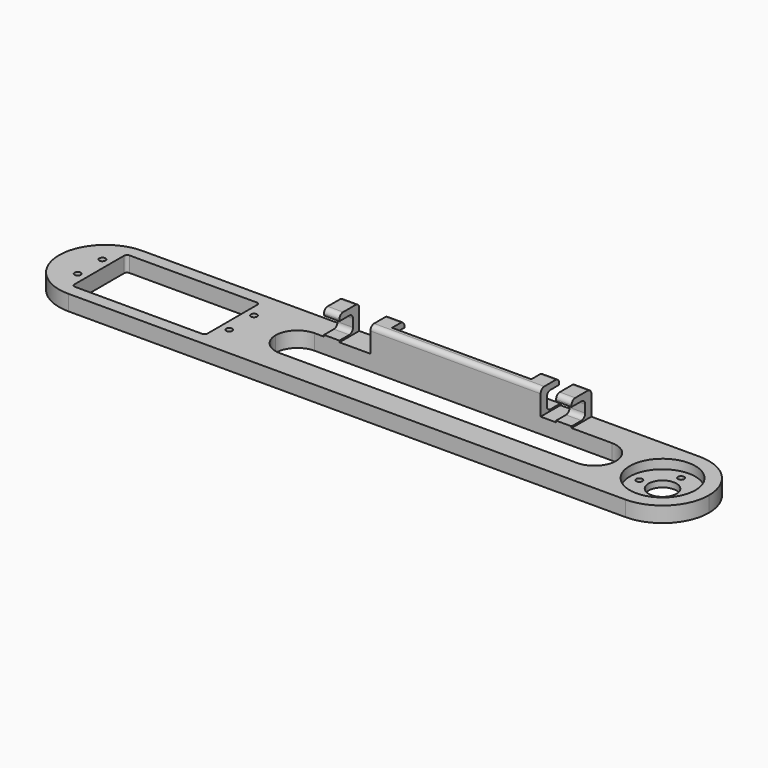
from build123d import *

# Parameters (mm, degrees)
F0_W      = 210
F0_H      = 30
F0_W_2    = 110
F0_H_2    = 14
F1_DEPTH  = 5
F2_R      = 10.6
F2_R_2    = 1
F2_R_3    = 4.5
F2_W      = 43
F2_H      = 22
F2_R_4    = 2.75
F3_DEPTH  = 3
F4_DEPTH  = 25
F5_R      = 14.99999
F6_R      = 6.99999
F7_R      = 1
F8_DEPTH  = 25
F9_W      = 5
F9_H      = 8
F10_DEPTH = 8
F11_W     = 5.5
F11_H     = 5.5
F12_DEPTH = 6
F13_W     = 5.5
F13_H     = 5.5
F14_DEPTH = 6
F15_W     = 5.5
F15_H     = 5.5
F16_W     = 5.5
F16_H     = 5.5
F17_DEPTH = 6
F9_W_2    = 45
F9_H_2    = 2.5
F18_DEPTH = 8
F19_DEPTH = 0.5
F20_R     = 1.5


# Not quite as in the source:
# - a fillet or chamfer is up to 0.001 mm smaller than in the source, because OpenCascade refuses the exact size
# - a feature names something its author has since deleted; it is built from what else it names


with BuildPart() as f1:
    # F0 (on Top) → F1 (new body)
    with BuildSketch(Plane.XY):
        with Locations((-5, -11.8972941886)):
            Rectangle(F0_W, F0_H)
        with Locations((15, -11.8972941886)):
            Rectangle(F0_W_2, F0_H_2, mode=Mode.SUBTRACT)
    extrude(amount=F1_DEPTH)

    # F2 (on face) → F3 (cut)
    with BuildSketch(Plane.XY.offset(5)):
        with Locations((85, -11.8972941886)):
            Circle(F2_R)
        with Locations((85, -19.3972941886)):
            Circle(F2_R_2, mode=Mode.SUBTRACT)
        with Locations((85, -11.8972941886)):
            Circle(F2_R_3, mode=Mode.SUBTRACT)
        with Locations((77.5, -11.8972941886)):
            Circle(F2_R_2, mode=Mode.SUBTRACT)
        with Locations((92.5, -11.8972941886)):
            Circle(F2_R_2, mode=Mode.SUBTRACT)
        with Locations((85, -4.3972941886)):
            Circle(F2_R_2, mode=Mode.SUBTRACT)
        with Locations((-75.5, -11.8972941886)):
            Rectangle(F2_W, F2_H)
        with Locations((-65, -11.8972941886)):
            Circle(F2_R_4, mode=Mode.SUBTRACT)
    extrude(amount=-F3_DEPTH, mode=Mode.SUBTRACT)

    # F2 (on face) → F4 (cut)
    with BuildSketch(Plane.XY.offset(5)):
        with Locations((-75.5, -11.8972941886)):
            Rectangle(F2_W, F2_H)
        with Locations((-65, -11.8972941886)):
            Circle(F2_R_4, mode=Mode.SUBTRACT)
        with Locations((85, -11.8972941886)):
            Circle(F2_R_3)
        with Locations((-65, -11.8972941886)):
            Circle(F2_R_4)
        with Locations((85, -4.3972941886)):
            Circle(F2_R_2)
        with Locations((77.5, -11.8972941886)):
            Circle(F2_R_2)
        with Locations((85, -19.3972941886)):
            Circle(F2_R_2)
        with Locations((92.5, -11.8972941886)):
            Circle(F2_R_2)
    extrude(amount=-F4_DEPTH, mode=Mode.SUBTRACT)

    # F5 (radius 15 in the source; OpenCascade refuses exactly that, so slightly less here)
    f5_edges = [f1.edges().sort_by_distance(p)[0] for p in [
        (100, 3.102706, 2.5),
        (100, -26.897294, 2.5),
        (-110, -26.897294, 2.5),
        (-110, 3.102706, 2.5),
    ]]
    fillet(f5_edges, radius=F5_R)

    # F6 (radius 7 in the source; OpenCascade refuses exactly that, so slightly less here)
    f6_edges = [f1.edges().sort_by_distance(p)[0] for p in [
        (-40, -4.897294, 2.5),
        (-40, -18.897294, 2.5),
        (70, -4.897294, 2.5),
        (70, -18.897294, 2.5),
    ]]
    fillet(f6_edges, radius=F6_R)

    # F7
    f7_edges = [f1.edges().sort_by_distance(p)[0] for p in [
        (-97, -0.897294, 2.5),
        (-97, -22.897294, 2.5),
        (-54, -0.897294, 2.5),
        (-54, -22.897294, 2.5),
    ]]
    fillet(f7_edges, radius=F7_R)

    # F2 (on face) → F8 (cut)
    with BuildSketch(Plane.XY.offset(5)):
        with Locations((-100, -6.8972941886)):
            Circle(F2_R_2)
        with Locations((-100, -16.8972941886)):
            Circle(F2_R_2)
        with Locations((-51, -6.8972941886)):
            Circle(F2_R_2)
        with Locations((-51, -16.8972941886)):
            Circle(F2_R_2)
    extrude(amount=-F8_DEPTH, mode=Mode.SUBTRACT)

    # F9 (on face) → F10 (join)
    with BuildSketch(Plane.XY.offset(5)):
        with Locations((-27.5, -0.8972941886)):
            Rectangle(F9_W, F9_H)
        Polygon((-10, 3.1027058114), (-15, 3.1027058114), (-15, -4.8972941886), (-10, -4.8972941886), (-10, -2.3972941886), align=None)
        Polygon((40, 3.1027058114), (35, 3.1027058114), (35, -2.3972941886), (35, -4.8972941886), (40, -4.8972941886), align=None)
        with Locations((47.5, -0.8972941886)):
            Rectangle(F9_W, F9_H)
    extrude(amount=F10_DEPTH)

    # F11 (on face) → F12 (cut)
    with BuildSketch(Plane(origin=(-30, 0, 0), x_dir=(0, -1, 0), z_dir=(-1, 0, 0))):
        with Locations((2.1472941886, 8.25)):
            Rectangle(F11_W, F11_H)
    extrude(amount=-F12_DEPTH, mode=Mode.SUBTRACT)

    # F13 (on face) → F14 (cut)
    with BuildSketch(Plane(origin=(-15, 0, 0), x_dir=(0, -1, 0), z_dir=(-1, 0, 0))):
        with Locations((-0.3527058114, 8.25)):
            Rectangle(F13_W, F13_H)
    extrude(amount=-F14_DEPTH, mode=Mode.SUBTRACT)

    # F15 (on face) + F16 (on face) → F17 (cut)
    with BuildSketch(Plane(origin=(35, 0, 0), x_dir=(0, -1, 0), z_dir=(-1, 0, 0))):
        with Locations((-0.3527058114, 8.25)):
            Rectangle(F15_W, F15_H)
    with BuildSketch(Plane(origin=(45, 0, 0), x_dir=(0, -1, 0), z_dir=(-1, 0, 0))):
        with Locations((2.1472941886, 8.25)):
            Rectangle(F16_W, F16_H)
    extrude(amount=-F17_DEPTH, mode=Mode.SUBTRACT)

    # F9 (on face) → F18 (join)
    with BuildSketch(Plane.XY.offset(5)):
        with Locations((12.5, -3.6472941886)):
            Rectangle(F9_W_2, F9_H_2)
    extrude(amount=F18_DEPTH)

    # F19 (cut): faces of the model
    f19_faces = [f1.faces().sort_by_distance(p)[0] for p in [
        (37.5, 3.1027058114, 12),
        (-12.5, 3.1027058114, 12),
        (47.5, -4.8972941886, 12),
        (-27.5, -4.8972941886, 12),
    ]]
    extrude(f19_faces, amount=-F19_DEPTH, dir=(0, 1, 0), mode=Mode.SUBTRACT)

    # F20
    f20_edges = [f1.edges().sort_by_distance(p)[0] for p in [
        (-27.5, 3.102706, 13),
        (-27.5, -4.897294, 13),
        (12.5, -4.897294, 13),
        (-12.5, 2.602706, 13),
        (-12.5, -2.397294, 5.5),
        (-12.5, -2.397294, 11),
        (-27.5, 0.602706, 5.5),
        (-27.5, 0.602706, 11),
        (37.5, 2.602706, 13),
        (47.5, 3.102706, 13),
        (47.5, -4.897294, 13),
        (37.5, -2.397294, 11),
        (37.5, -2.397294, 5.5),
        (47.5, 0.602706, 5.5),
        (47.5, 0.602706, 11),
    ]]
    fillet(f20_edges, radius=F20_R)


solid = f1.part
